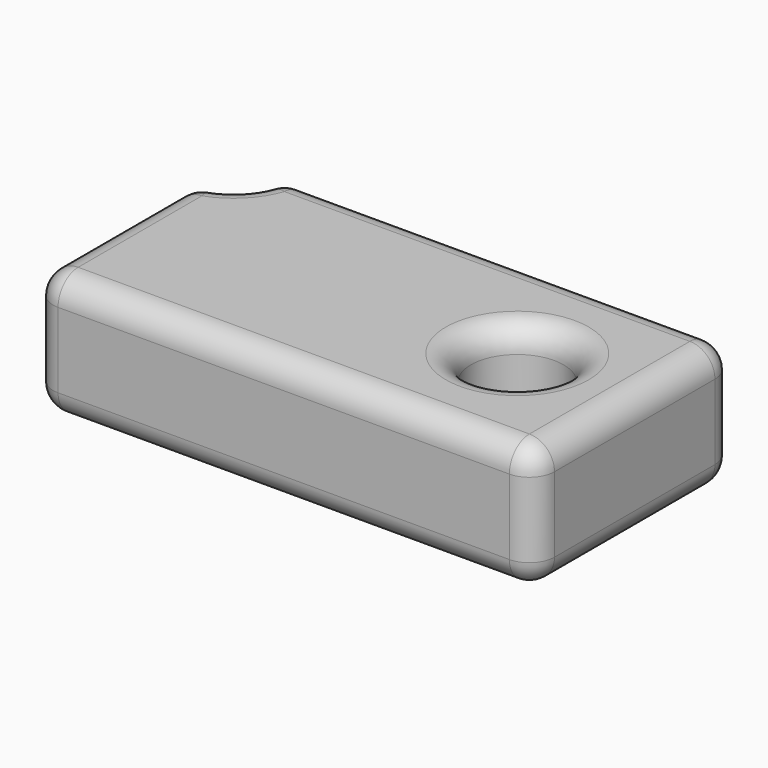
from build123d import *

# Parameters (mm, degrees)
F0_R     = 9.2551404176
F1_DEPTH = 25
F3_F1_R  = 5
F3_F2_R  = 5
F3_F3_R  = 5
F3_F4_R  = 5
F3_F5_R  = 5
F3_F6_R  = 5
F3_F7_R  = 5
F3_F8_R  = 5
F3_F9_R  = 5


# Not quite as in the source:
# - a feature of the source that left no trace in its solid (it failed there, or was rolled back) is left out


with BuildPart() as f1:
    # F0 (on Top) → F1 (new body)
    with BuildSketch(Plane.XY):
        with BuildLine():
            Line((50, -25), (50, 25))
            Line((50, 25), (-40, 25))
            ThreePointArc((-40, 25), (-42.9289321881, 17.9289321881), (-50, 15))
            Line((-50, 15), (-50, -25))
            Line((-50, -25), (50, -25))
        make_face()
        with Locations((26.5483168381, 0.0399786921)):
            Circle(F0_R, mode=Mode.SUBTRACT)
    extrude(amount=F1_DEPTH)

    # F3: fillet of radius 5 on 15 edges, made by hand

    # F3_f1
    f3_f1_edges = [f1.edges().sort_by_distance(p)[0] for p in [
        (-50, 15, 12.5),
    ]]
    fillet(f3_f1_edges, radius=F3_F1_R)

    # F3_f2
    f3_f2_edges = [f1.edges().sort_by_distance(p)[0] for p in [
        (-50, -25, 12.5),
    ]]
    fillet(f3_f2_edges, radius=F3_F2_R)

    # F3_f3
    f3_f3_edges = [f1.edges().sort_by_distance(p)[0] for p in [
        (50, -25, 12.5),
    ]]
    fillet(f3_f3_edges, radius=F3_F3_R)

    # F3_f4
    f3_f4_edges = [f1.edges().sort_by_distance(p)[0] for p in [
        (50, 25, 12.5),
    ]]
    fillet(f3_f4_edges, radius=F3_F4_R)

    # F3_f5
    f3_f5_edges = [f1.edges().sort_by_distance(p)[0] for p in [
        (-40, 25, 12.5),
    ]]
    fillet(f3_f5_edges, radius=F3_F5_R)

    # F3_f6
    f3_f6_edges = [f1.edges().sort_by_distance(p)[0] for p in [
        (-50, -4.5710678119, 0),
    ]]
    fillet(f3_f6_edges, radius=F3_F6_R)

    # F3_f7
    f3_f7_edges = [f1.edges().sort_by_distance(p)[0] for p in [
        (-50, -4.5710678119, 25),
    ]]
    fillet(f3_f7_edges, radius=F3_F7_R)

    # F3_f8
    f3_f8_edges = [f1.edges().sort_by_distance(p)[0] for p in [
        (17.2931764204, 0.0399786921, 0),
    ]]
    fillet(f3_f8_edges, radius=F3_F8_R)

    # F3_f9
    f3_f9_edges = [f1.edges().sort_by_distance(p)[0] for p in [
        (17.2931764204, 0.0399786921, 25),
    ]]
    fillet(f3_f9_edges, radius=F3_F9_R)


solid = f1.part
